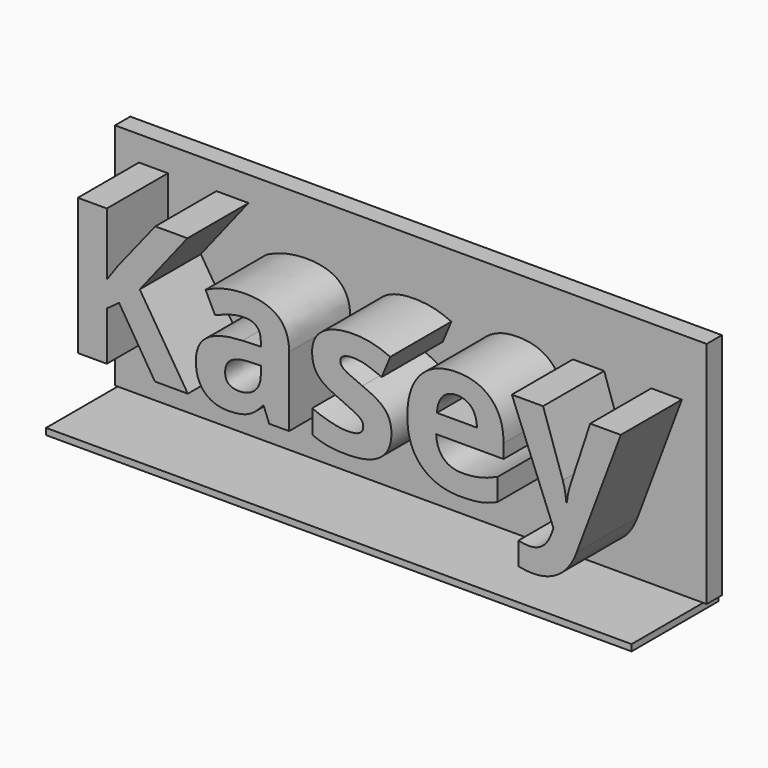
from build123d import *

# Parameters (mm, degrees)
F1_W         = 155
F1_H         = 60
F2_DEPTH     = 5
F0_TEXT_SIZE = 50.1724678583
F3_DEPTH     = 25
F4_W         = 153.3874720335
F4_H         = 1.68866897
F5_DEPTH     = 28.448


# Not quite as in the source:
# - Text() gives the source's letters only with a copy of the font that has no kerning and outlines rounded to 1/6400 em; it was checked with that copy


with BuildPart() as f2:
    # F1 (on Front) → F2 (new body)
    with BuildSketch(Plane.XZ):
        with Locations((0.7391198714, 25.3300438635)):
            Rectangle(F1_W, F1_H)
    extrude(amount=F2_DEPTH)

    # F0 (on Front) → F3 (join)
    with BuildSketch(Plane.XZ):
        with Locations((-75, 12.9821116747)):
            Text('Kasey', F0_TEXT_SIZE, font='Open Sans', font_style=FontStyle.BOLD, text_align=(TextAlign.LEFT, TextAlign.BOTTOM))
    extrude(amount=F3_DEPTH)

    # F4 (on Front) → F5 (join)
    with BuildSketch(Plane.XZ):
        with Locations((0.6360858679, -5.5142906215)):
            Rectangle(F4_W, F4_H)
    extrude(amount=F5_DEPTH)


solid = f2.part
